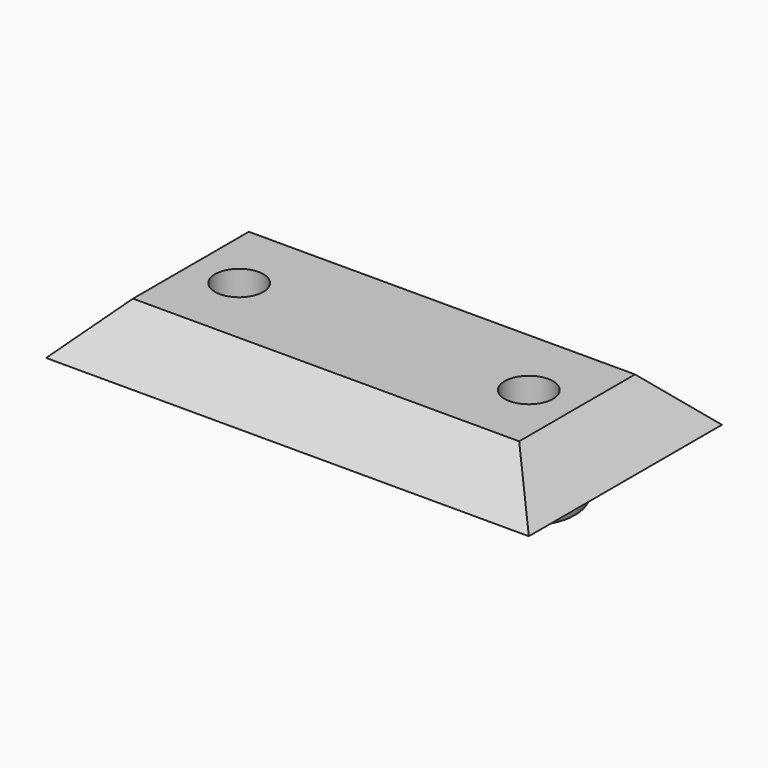
from build123d import *

# Parameters (mm, degrees)
F0_R     = 6.35
F0_R_2   = 3.175
F1_DEPTH = 6.35
F2_SIZE  = 6.34999
F3_DEPTH = 6.351
F4_DEPTH = 6.35
F5_R     = 0.7939024


# Not quite as in the source:
# - a fillet or chamfer is up to 0.001 mm smaller than in the source, because OpenCascade refuses the exact size


with BuildPart() as f1:
    # F0 (on Top) → F1 (new body)
    with BuildSketch(Plane.XY):
        Polygon((-14.2875, 15.875), (-23.8125, 15.875), (-23.8125, 7.9375), (-31.75, 7.9375), (-31.75, -7.9375), (-23.8125, -7.9375), (-23.8125, -15.875), (-14.2875, -15.875), (-14.2875, -7.9375), (-6.35, -7.9375), (-6.35, -15.875), (6.35, -15.875), (6.35, -7.9375), (14.2875, -7.9375), (14.2875, -15.875), (23.8125, -15.875), (23.8125, -7.9375), (31.75, -7.9375), (31.75, 7.9375), (23.8125, 7.9375), (23.8125, 15.875), (14.2875, 15.875), (14.2875, 7.9375), (6.35, 7.9375), (6.35, 15.875), (-6.35, 15.875), (-6.35, 7.9375), (-14.2875, 7.9375), align=None)
        with Locations((-19.05, 0)):
            Circle(F0_R, mode=Mode.SUBTRACT)
        with Locations((19.05, 0)):
            Circle(F0_R, mode=Mode.SUBTRACT)
        with Locations((-19.05, 0)):
            Circle(F0_R)
        with Locations((-19.05, 0)):
            Circle(F0_R_2, mode=Mode.SUBTRACT)
        with Locations((19.05, 0)):
            Circle(F0_R)
        with Locations((19.05, 0)):
            Circle(F0_R_2, mode=Mode.SUBTRACT)
        with Locations((-19.05, 0)):
            Circle(F0_R_2)
        with Locations((19.05, 0)):
            Circle(F0_R_2)
        Polygon((-23.8125, 7.9375), (-31.75, 15.875), (-31.75, 7.9375), align=None)
        Polygon((-23.8125, 15.875), (-31.75, 15.875), (-23.8125, 7.9375), align=None)
        Polygon((-6.35, 15.875), (-14.2875, 15.875), (-14.2875, 7.9375), align=None)
        Polygon((-6.35, 7.9375), (-6.35, 15.875), (-14.2875, 7.9375), align=None)
        Polygon((14.2875, 7.9375), (6.35, 15.875), (6.35, 7.9375), align=None)
        Polygon((14.2875, 15.875), (6.35, 15.875), (14.2875, 7.9375), align=None)
        Polygon((31.75, 15.875), (23.8125, 15.875), (23.8125, 7.9375), align=None)
        Polygon((31.75, 7.9375), (31.75, 15.875), (23.8125, 7.9375), align=None)
        Polygon((31.75, -15.875), (31.75, -7.9375), (23.8125, -7.9375), align=None)
        Polygon((23.8125, -7.9375), (23.8125, -15.875), (31.75, -15.875), align=None)
        Polygon((14.2875, -7.9375), (6.35, -15.875), (14.2875, -15.875), align=None)
        Polygon((6.35, -7.9375), (6.35, -15.875), (14.2875, -7.9375), align=None)
        Polygon((-14.2875, -7.9375), (-6.35, -15.875), (-6.35, -7.9375), align=None)
        Polygon((-14.2875, -7.9375), (-14.2875, -15.875), (-6.35, -15.875), align=None)
        Polygon((-23.8125, -7.9375), (-31.75, -15.875), (-23.8125, -15.875), align=None)
        Polygon((-23.8125, -7.9375), (-31.75, -7.9375), (-31.75, -15.875), align=None)
    extrude(amount=F1_DEPTH)

    # F2 (size 6.35 in the source; OpenCascade refuses exactly that, so slightly less here)
    f2_edges = [f1.edges().sort_by_distance(p)[0] for p in [
        (31.75, 0, 6.35),
        (0, 15.875, 6.35),
        (-31.75, 0, 6.35),
        (0, -15.875, 6.35),
    ]]
    chamfer(f2_edges, length=F2_SIZE)

    # F0 (on Top) → F3 (cut, through all)
    with BuildSketch(Plane.XY):
        with Locations((-19.05, 0)):
            Circle(F0_R_2)
        with Locations((19.05, 0)):
            Circle(F0_R_2)
    extrude(amount=F3_DEPTH, mode=Mode.SUBTRACT)

    # F0 (on Top) → F4 (join)
    with BuildSketch(Plane.XY):
        with Locations((-19.05, 0)):
            Circle(F0_R)
        with Locations((-19.05, 0)):
            Circle(F0_R_2, mode=Mode.SUBTRACT)
        with Locations((19.05, 0)):
            Circle(F0_R)
        with Locations((19.05, 0)):
            Circle(F0_R_2, mode=Mode.SUBTRACT)
    extrude(amount=-F4_DEPTH)

    # F5
    f5_edges = [f1.edges().sort_by_distance(p)[0] for p in [
        (-25.4, 0, -6.35),
        (12.7, 0, -6.35),
    ]]
    fillet(f5_edges, radius=F5_R)


solid = f1.part
